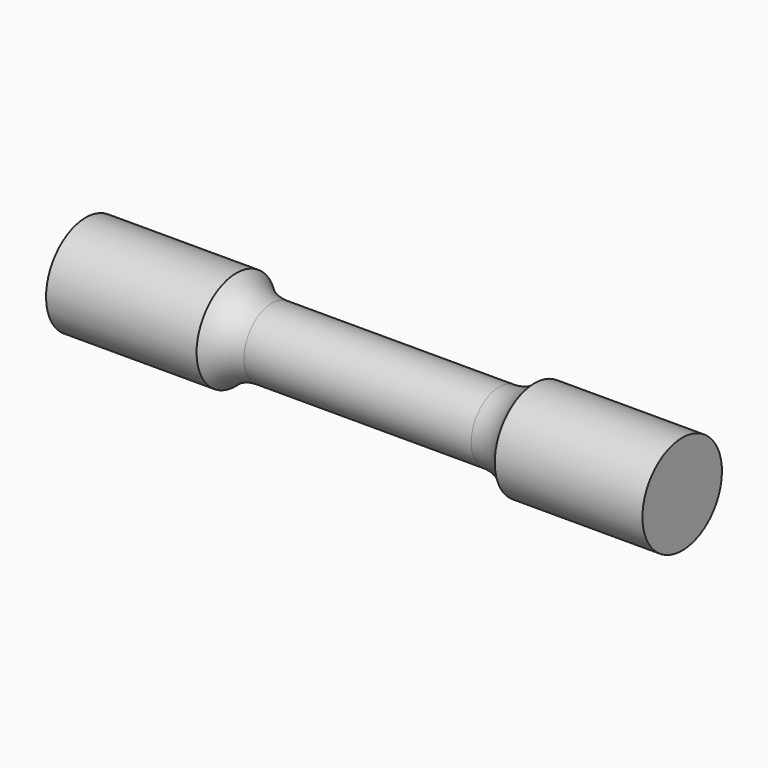
from build123d import *

# Parameters (mm, degrees)
F0_W = 1524
F0_H = 127
F2_W = 762
F2_H = 305.5362462927


# Not quite as in the source:
# - a fillet or chamfer that OpenCascade refuses, or shapes differently, is made with other operations: its cross-section is extruded or revolved along the edge and cut away or added


with BuildPart() as f1:
    # F0 (on Front) → F1 (revolve)
    with BuildSketch(Plane.XZ):
        with Locations((128.8676711868, 63.5)):
            Rectangle(F0_W, F0_H)
    revolve(axis=Axis((128.8676711868, 0, 0), (1, 0, 0)))

    # F2 (on Front) → F3 (revolve, cut)
    with BuildSketch(Plane.XZ):
        with Locations((132.5217391304, 241.6681231464)):
            Rectangle(F2_W, F2_H)
    revolve(axis=Axis((22.0869673282, 0, 0), (1, 0, 0)), mode=Mode.SUBTRACT)

    # F4: fillet of radius 127 on 1 edges, made by hand

    # F4_s1 → F4_t2 (revolve)
    with BuildSketch(Plane.XZ):
        with BuildLine():
            ThreePointArc((-248.4782608696, 127), (-206.9690083239, 98.8117853924), (-157.7821198271, 88.9))
            Line((-157.7821198271, 88.9), (-248.4782608696, 88.9))
            Line((-248.4782608696, 88.9), (-248.4782608696, 127))
        make_face()
    revolve(axis=Axis((-248.4782608696, 0, 0), (1, 0, 0)))

    # F5: fillet of radius 127 on 1 edges, made by hand

    # F5_s1 → F5_t2 (revolve)
    with BuildSketch(Plane.XZ):
        with BuildLine():
            ThreePointArc((422.8255980879, 88.9), (472.0124865848, 98.8117853924), (513.5217391304, 127))
            Line((513.5217391304, 127), (513.5217391304, 88.9))
            Line((513.5217391304, 88.9), (422.8255980879, 88.9))
        make_face()
    revolve(axis=Axis((513.5217391304, 0, 0), (1, 0, 0)))


solid = f1.part
